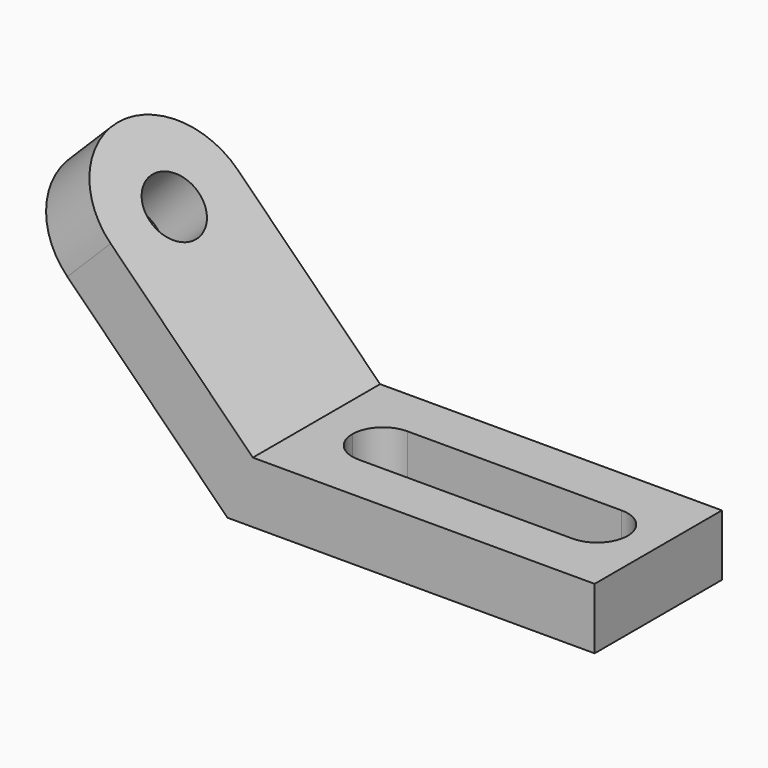
from build123d import *

# Parameters (mm, degrees)
F0_W     = 90
F0_H     = 20
F0_W_2   = 10
F1_DEPTH = 52
F2_R     = 25.99999
F4_DEPTH = 25
F6_DEPTH = 25


# Not quite as in the source:
# - a fillet or chamfer is up to 0.001 mm smaller than in the source, because OpenCascade refuses the exact size


with BuildPart() as f1:
    # F0 (on Front) → F1 (new body)
    with BuildSketch(Plane.XZ):
        Polygon((-45.2548339959, 45.2548339959), (0, 0), (20, 0), (20, 20), (8.2842712475, 20), (-31.1126983722, 59.3969696197), align=None)
        with Locations((65, 10)):
            Rectangle(F0_W, F0_H)
        Polygon((-59.3969696197, 59.3969696197), (-45.2548339959, 45.2548339959), (-31.1126983722, 59.3969696197), (-45.2548339959, 73.5391052434), align=None)
        with Locations((115, 10)):
            Rectangle(F0_W_2, F0_H)
        Polygon((-70.7106781187, 70.7106781187), (-59.3969696197, 59.3969696197), (-45.2548339959, 73.5391052434), (-56.5685424949, 84.8528137424), align=None)
    extrude(amount=F1_DEPTH)

    # F2 (radius 26 in the source; OpenCascade refuses exactly that, so slightly less here)
    f2_edges = [f1.edges().sort_by_distance(p)[0] for p in [
        (-63.63961, 0, 77.781746),
        (-63.63961, -52, 77.781746),
    ]]
    fillet(f2_edges, radius=F2_R)

    # F3 (on face) → F4 (cut)
    with BuildSketch(Plane(origin=(14.1421356237, 0, 14.1421356237), x_dir=(0.7071067812, 0, -0.7071067812), z_dir=(0.7071067812, 0, 0.7071067812))):
        with BuildLine():
            ThreePointArc((-84, -26), (-74, -36), (-64, -26))
            ThreePointArc((-64, -26), (-74, -16), (-84, -26))
        make_face()
    extrude(amount=-F4_DEPTH, mode=Mode.SUBTRACT)

    # F5 (on face) → F6 (cut)
    with BuildSketch(Plane.XY.offset(20)):
        with BuildLine():
            Line((100, -16), (30, -16))
            ThreePointArc((30, -16), (22.9289321881, -18.9289321881), (20, -26))
            ThreePointArc((20, -26), (22.9289321881, -33.0710678119), (30, -36))
            Line((30, -36), (100, -36))
            ThreePointArc((100, -36), (107.0710678119, -33.0710678119), (110, -26))
            ThreePointArc((110, -26), (107.0710678119, -18.9289321881), (100, -16))
        make_face()
    extrude(amount=-F6_DEPTH, mode=Mode.SUBTRACT)


solid = f1.part
